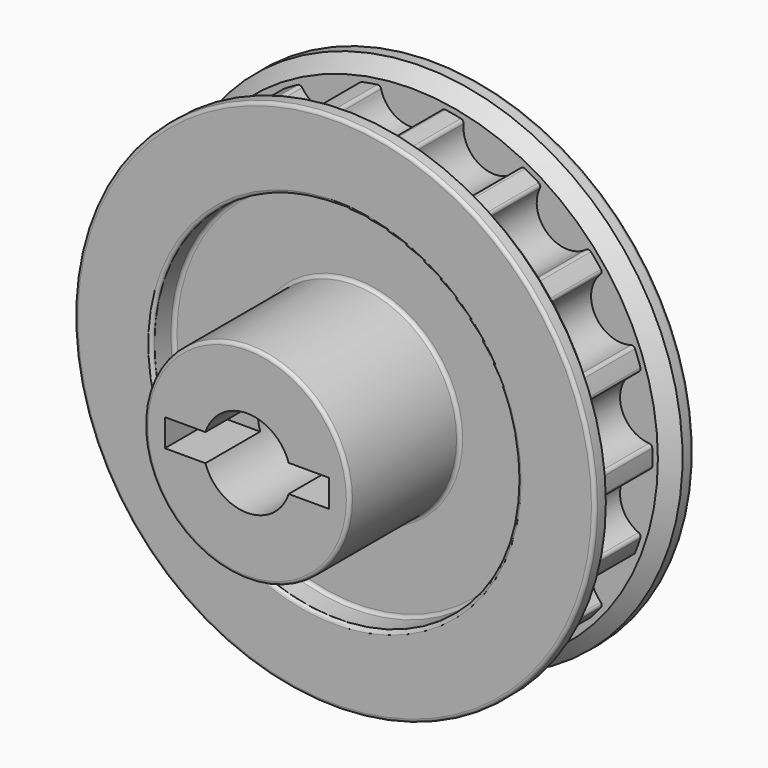
from build123d import *

# Parameters (mm, degrees)
F0_R      = 20.2099238274
F0_R_2    = 2.2772854034
F1_DEPTH  = 5
F2_R      = 21.3644414185
F2_R_2    = 17.5995160556
F3_DEPTH  = 5
F4_R      = 19
F4_R_2    = 13.3671533493
F5_DEPTH  = 2
F6_SIZE2  = 1
F6_SIZE   = 1
F7_R      = 19
F7_R_2    = 13.3703320349
F8_DEPTH  = 2
F9_SIZE2  = 1
F9_SIZE   = 1
F10_R     = 7.5
F11_DEPTH = 10
F12_R     = 3.2
F13_DEPTH = 15
F15_DEPTH = 5
F16_R     = 0.25


# Not quite as in the source:
# - two fillets or chamfers of one size are made in one step


with BuildPart() as f1:
    # F0 (on Front) → F1 (new body)
    with BuildSketch(Plane.XZ):
        with Locations((-33.3708077669, 18.9050808549)):
            Circle(F0_R)
        with Locations((-44.8001539134, 5.2841165238)):
            Circle(F0_R_2, mode=Mode.SUBTRACT)
        with Locations((-39.4522358284, 2.1964945778)):
            Circle(F0_R_2, mode=Mode.SUBTRACT)
        with Locations((-48.7695241739, 10.0146277921)):
            Circle(F0_R_2, mode=Mode.SUBTRACT)
        with Locations((-50.8815819749, 15.8174589089)):
            Circle(F0_R_2, mode=Mode.SUBTRACT)
        with Locations((-33.3708077669, 1.1241747293)):
            Circle(F0_R_2, mode=Mode.SUBTRACT)
        with Locations((-27.2893797054, 2.1964945778)):
            Circle(F0_R_2, mode=Mode.SUBTRACT)
        with Locations((-21.9414616204, 5.2841165238)):
            Circle(F0_R_2, mode=Mode.SUBTRACT)
        with Locations((-17.9720913599, 10.0146277921)):
            Circle(F0_R_2, mode=Mode.SUBTRACT)
        with Locations((-15.8600335589, 15.8174589089)):
            Circle(F0_R_2, mode=Mode.SUBTRACT)
        with Locations((-50.8815819749, 21.9927028009)):
            Circle(F0_R_2, mode=Mode.SUBTRACT)
        with Locations((-48.7695241739, 27.7955339177)):
            Circle(F0_R_2, mode=Mode.SUBTRACT)
        with Locations((-44.8001539134, 32.526045186)):
            Circle(F0_R_2, mode=Mode.SUBTRACT)
        with Locations((-39.4522358284, 35.613667132)):
            Circle(F0_R_2, mode=Mode.SUBTRACT)
        with Locations((-33.3708077669, 36.6859869804)):
            Circle(F0_R_2, mode=Mode.SUBTRACT)
        with Locations((-15.8600335589, 21.9927028009)):
            Circle(F0_R_2, mode=Mode.SUBTRACT)
        with Locations((-17.9720913599, 27.7955339177)):
            Circle(F0_R_2, mode=Mode.SUBTRACT)
        with Locations((-27.2893797054, 35.613667132)):
            Circle(F0_R_2, mode=Mode.SUBTRACT)
        with Locations((-21.9414616204, 32.526045186)):
            Circle(F0_R_2, mode=Mode.SUBTRACT)
    extrude(amount=F1_DEPTH)

    # F2 (on face) → F3 (cut)
    with BuildSketch(Plane.XZ.offset(5)):
        with Locations((-33.3708077669, 18.9050808549)):
            Circle(F2_R)
        with Locations((-33.3708077669, 18.9050808549)):
            Circle(F2_R_2, mode=Mode.SUBTRACT)
    extrude(amount=-F3_DEPTH, mode=Mode.SUBTRACT)

    # F4 (on face) → F5 (join)
    with BuildSketch(Plane.XZ.offset(5)):
        with Locations((-33.3708077669, 18.9050808549)):
            Circle(F4_R)
        with BuildLine():
            ThreePointArc((-46.3169163653, 6.982780844), (-46.8528192429, 7.5923299979), (-47.3600494173, 8.2259384063))
            ThreePointArc((-47.3600494173, 8.2259384063), (-46.797337163, 11.1532704938), (-49.6138372432, 12.1296134302))
            ThreePointArc((-49.6138372432, 12.1296134302), (-49.9089431338, 12.8856918511), (-50.1688767471, 13.654571934))
            ThreePointArc((-50.1688767471, 13.654571934), (-48.6388936539, 16.2129053692), (-50.9516090447, 18.0936673831))
            ThreePointArc((-50.9516090447, 18.0936673831), (-50.9703238225, 18.9050808549), (-50.9516090447, 19.7164943267))
            ThreePointArc((-50.9516090447, 19.7164943267), (-48.6388936539, 21.5972563405), (-50.1688767471, 24.1555897758))
            ThreePointArc((-50.1688767471, 24.1555897758), (-49.9089431338, 24.9244698587), (-49.6138372432, 25.6805482796))
            ThreePointArc((-49.6138372432, 25.6805482796), (-46.797337163, 26.656891216), (-47.3600494173, 29.5842233035))
            ThreePointArc((-47.3600494173, 29.5842233035), (-46.8528192429, 30.2178317119), (-46.3169163653, 30.8273808658))
            ThreePointArc((-46.3169163653, 30.8273808658), (-43.3363430724, 30.7815433574), (-42.8639130854, 33.7247946444))
            ThreePointArc((-42.8639130854, 33.7247946444), (-42.1705657947, 34.1467088533), (-41.4585037262, 34.5362081162))
            ThreePointArc((-41.4585037262, 34.5362081162), (-38.6733583484, 33.473718843), (-37.2227681487, 36.0778897867))
            ThreePointArc((-37.2227681487, 36.0778897867), (-36.4269316578, 36.2372207157), (-35.6245955928, 36.3596907281))
            ThreePointArc((-35.6245955928, 36.3596907281), (-33.3708077669, 34.4087015771), (-31.117019941, 36.3596907281))
            ThreePointArc((-31.117019941, 36.3596907281), (-30.314683876, 36.2372207157), (-29.5188473852, 36.0778897867))
            ThreePointArc((-29.5188473852, 36.0778897867), (-28.0682571854, 33.473718843), (-25.2831118076, 34.5362081162))
            ThreePointArc((-25.2831118076, 34.5362081162), (-24.5710497391, 34.1467088533), (-23.8777024485, 33.7247946444))
            ThreePointArc((-23.8777024485, 33.7247946444), (-23.4052724614, 30.7815433574), (-20.4246991685, 30.8273808658))
            ThreePointArc((-20.4246991685, 30.8273808658), (-19.8887962909, 30.2178317119), (-19.3815661165, 29.5842233035))
            ThreePointArc((-19.3815661165, 29.5842233035), (-19.9442783709, 26.656891216), (-17.1277782906, 25.6805482796))
            ThreePointArc((-17.1277782906, 25.6805482796), (-16.8326724001, 24.9244698587), (-16.5727387868, 24.1555897758))
            ThreePointArc((-16.5727387868, 24.1555897758), (-18.1027218799, 21.5972563405), (-15.7900064891, 19.7164943267))
            ThreePointArc((-15.7900064891, 19.7164943267), (-15.7712917113, 18.9050808549), (-15.7900064891, 18.0936673831))
            ThreePointArc((-15.7900064891, 18.0936673831), (-18.1027218799, 16.2129053692), (-16.5727387868, 13.654571934))
            ThreePointArc((-16.5727387868, 13.654571934), (-16.8326724001, 12.8856918511), (-17.1277782906, 12.1296134302))
            ThreePointArc((-17.1277782906, 12.1296134302), (-19.9442783709, 11.1532704938), (-19.3815661165, 8.2259384063))
            ThreePointArc((-19.3815661165, 8.2259384063), (-19.8887962909, 7.5923299979), (-20.4246991685, 6.982780844))
            ThreePointArc((-20.4246991685, 6.982780844), (-23.4052724614, 7.0286183524), (-23.8777024485, 4.0853670654))
            ThreePointArc((-23.8777024485, 4.0853670654), (-24.5710497391, 3.6634528564), (-25.2831118076, 3.2739535935))
            ThreePointArc((-25.2831118076, 3.2739535935), (-28.0682571854, 4.3364428668), (-29.5188473852, 1.7322719231))
            ThreePointArc((-29.5188473852, 1.7322719231), (-30.314683876, 1.5729409941), (-31.117019941, 1.4504709817))
            ThreePointArc((-31.117019941, 1.4504709817), (-33.3708077669, 3.4014601327), (-35.6245955928, 1.4504709817))
            ThreePointArc((-35.6245955928, 1.4504709817), (-36.4269316578, 1.5729409941), (-37.2227681487, 1.7322719231))
            ThreePointArc((-37.2227681487, 1.7322719231), (-38.6733583484, 4.3364428668), (-41.4585037262, 3.2739535935))
            ThreePointArc((-41.4585037262, 3.2739535935), (-42.1705657947, 3.6634528564), (-42.8639130854, 4.0853670654))
            ThreePointArc((-42.8639130854, 4.0853670654), (-43.3363430724, 7.0286183524), (-46.3169163653, 6.982780844))
        make_face(mode=Mode.SUBTRACT)
        with BuildLine():
            ThreePointArc((-49.6138372432, 12.1296134302), (-46.797337163, 11.1532704938), (-47.3600494173, 8.2259384063))
            ThreePointArc((-47.3600494173, 8.2259384063), (-46.8528192429, 7.5923299979), (-46.3169163653, 6.982780844))
            ThreePointArc((-46.3169163653, 6.982780844), (-43.3363430724, 7.0286183524), (-42.8639130854, 4.0853670654))
            ThreePointArc((-42.8639130854, 4.0853670654), (-42.1705657947, 3.6634528564), (-41.4585037262, 3.2739535935))
            ThreePointArc((-41.4585037262, 3.2739535935), (-38.6733583484, 4.3364428668), (-37.2227681487, 1.7322719231))
            ThreePointArc((-37.2227681487, 1.7322719231), (-36.4269316578, 1.5729409941), (-35.6245955928, 1.4504709817))
            ThreePointArc((-35.6245955928, 1.4504709817), (-33.3708077669, 3.4014601327), (-31.117019941, 1.4504709817))
            ThreePointArc((-31.117019941, 1.4504709817), (-30.314683876, 1.5729409941), (-29.5188473852, 1.7322719231))
            ThreePointArc((-29.5188473852, 1.7322719231), (-28.0682571854, 4.3364428668), (-25.2831118076, 3.2739535935))
            ThreePointArc((-25.2831118076, 3.2739535935), (-24.5710497391, 3.6634528564), (-23.8777024485, 4.0853670654))
            ThreePointArc((-23.8777024485, 4.0853670654), (-23.4052724614, 7.0286183524), (-20.4246991685, 6.982780844))
            ThreePointArc((-20.4246991685, 6.982780844), (-19.8887962909, 7.5923299979), (-19.3815661165, 8.2259384063))
            ThreePointArc((-19.3815661165, 8.2259384063), (-19.9442783709, 11.1532704938), (-17.1277782906, 12.1296134302))
            ThreePointArc((-17.1277782906, 12.1296134302), (-16.8326724001, 12.8856918511), (-16.5727387868, 13.654571934))
            ThreePointArc((-16.5727387868, 13.654571934), (-18.1027218799, 16.2129053692), (-15.7900064891, 18.0936673831))
            ThreePointArc((-15.7900064891, 18.0936673831), (-15.7712917113, 18.9050808549), (-15.7900064891, 19.7164943267))
            ThreePointArc((-15.7900064891, 19.7164943267), (-18.1027218799, 21.5972563405), (-16.5727387868, 24.1555897758))
            ThreePointArc((-16.5727387868, 24.1555897758), (-16.8326724001, 24.9244698587), (-17.1277782906, 25.6805482796))
            ThreePointArc((-17.1277782906, 25.6805482796), (-19.9442783709, 26.656891216), (-19.3815661165, 29.5842233035))
            ThreePointArc((-19.3815661165, 29.5842233035), (-19.8887962909, 30.2178317119), (-20.4246991685, 30.8273808658))
            ThreePointArc((-20.4246991685, 30.8273808658), (-23.4052724614, 30.7815433574), (-23.8777024485, 33.7247946444))
            ThreePointArc((-23.8777024485, 33.7247946444), (-24.5710497391, 34.1467088533), (-25.2831118076, 34.5362081162))
            ThreePointArc((-25.2831118076, 34.5362081162), (-28.0682571854, 33.473718843), (-29.5188473852, 36.0778897867))
            ThreePointArc((-29.5188473852, 36.0778897867), (-30.314683876, 36.2372207157), (-31.117019941, 36.3596907281))
            ThreePointArc((-31.117019941, 36.3596907281), (-33.3708077669, 34.4087015771), (-35.6245955928, 36.3596907281))
            ThreePointArc((-35.6245955928, 36.3596907281), (-36.4269316578, 36.2372207157), (-37.2227681487, 36.0778897867))
            ThreePointArc((-37.2227681487, 36.0778897867), (-38.6733583484, 33.473718843), (-41.4585037262, 34.5362081162))
            ThreePointArc((-41.4585037262, 34.5362081162), (-42.1705657947, 34.1467088533), (-42.8639130854, 33.7247946444))
            ThreePointArc((-42.8639130854, 33.7247946444), (-43.3363430724, 30.7815433574), (-46.3169163653, 30.8273808658))
            ThreePointArc((-46.3169163653, 30.8273808658), (-46.8528192429, 30.2178317119), (-47.3600494173, 29.5842233035))
            ThreePointArc((-47.3600494173, 29.5842233035), (-46.797337163, 26.656891216), (-49.6138372432, 25.6805482796))
            ThreePointArc((-49.6138372432, 25.6805482796), (-49.9089431338, 24.9244698587), (-50.1688767471, 24.1555897758))
            ThreePointArc((-50.1688767471, 24.1555897758), (-48.6388936539, 21.5972563405), (-50.9516090447, 19.7164943267))
            ThreePointArc((-50.9516090447, 19.7164943267), (-50.9703238225, 18.9050808549), (-50.9516090447, 18.0936673831))
            ThreePointArc((-50.9516090447, 18.0936673831), (-48.6388936539, 16.2129053692), (-50.1688767471, 13.654571934))
            ThreePointArc((-50.1688767471, 13.654571934), (-49.9089431338, 12.8856918511), (-49.6138372432, 12.1296134302))
        make_face()
        with Locations((-33.3708077669, 18.9050808549)):
            Circle(F4_R_2, mode=Mode.SUBTRACT)
    extrude(amount=F5_DEPTH)

    # F6
    f6_edges = [f1.edges().sort_by_distance(p)[0] for p in [
        (-52.370808, -5, 18.905081),
    ]]
    chamfer(f6_edges, length=F6_SIZE, length2=F6_SIZE2)

    # F7 (on face) → F8 (join)
    with BuildSketch(Plane(origin=(0, 0, 0), x_dir=(-1, 0, 0), z_dir=(0, 1, 0))):
        with Locations((33.3708077669, 18.9050808549)):
            Circle(F7_R)
        with BuildLine():
            ThreePointArc((47.3600494173, 8.2259384063), (46.8528192429, 7.5923299979), (46.3169163653, 6.982780844))
            ThreePointArc((46.3169163653, 6.982780844), (43.3363430724, 7.0286183524), (42.8639130854, 4.0853670654))
            ThreePointArc((42.8639130854, 4.0853670654), (42.1705657947, 3.6634528564), (41.4585037262, 3.2739535935))
            ThreePointArc((41.4585037262, 3.2739535935), (38.6733583484, 4.3364428668), (37.2227681487, 1.7322719231))
            ThreePointArc((37.2227681487, 1.7322719231), (36.4269316578, 1.5729409941), (35.6245955928, 1.4504709817))
            ThreePointArc((35.6245955928, 1.4504709817), (33.3708077669, 3.4014601327), (31.117019941, 1.4504709817))
            ThreePointArc((31.117019941, 1.4504709817), (30.314683876, 1.5729409941), (29.5188473852, 1.7322719231))
            ThreePointArc((29.5188473852, 1.7322719231), (28.0682571854, 4.3364428668), (25.2831118076, 3.2739535935))
            ThreePointArc((25.2831118076, 3.2739535935), (24.5710497391, 3.6634528564), (23.8777024485, 4.0853670654))
            ThreePointArc((23.8777024485, 4.0853670654), (23.4052724614, 7.0286183524), (20.4246991685, 6.982780844))
            ThreePointArc((20.4246991685, 6.982780844), (19.8887962909, 7.5923299979), (19.3815661165, 8.2259384063))
            ThreePointArc((19.3815661165, 8.2259384063), (19.9442783709, 11.1532704938), (17.1277782906, 12.1296134302))
            ThreePointArc((17.1277782906, 12.1296134302), (16.8326724001, 12.8856918511), (16.5727387868, 13.654571934))
            ThreePointArc((16.5727387868, 13.654571934), (18.1027218799, 16.2129053692), (15.7900064891, 18.0936673831))
            ThreePointArc((15.7900064891, 18.0936673831), (15.7712917113, 18.9050808549), (15.7900064891, 19.7164943267))
            ThreePointArc((15.7900064891, 19.7164943267), (18.1027218799, 21.5972563405), (16.5727387868, 24.1555897758))
            ThreePointArc((16.5727387868, 24.1555897758), (16.8326724001, 24.9244698587), (17.1277782906, 25.6805482796))
            ThreePointArc((17.1277782906, 25.6805482796), (19.9442783709, 26.656891216), (19.3815661165, 29.5842233035))
            ThreePointArc((19.3815661165, 29.5842233035), (19.8887962909, 30.2178317119), (20.4246991685, 30.8273808658))
            ThreePointArc((20.4246991685, 30.8273808658), (23.4052724614, 30.7815433574), (23.8777024485, 33.7247946444))
            ThreePointArc((23.8777024485, 33.7247946444), (24.5710497391, 34.1467088533), (25.2831118076, 34.5362081162))
            ThreePointArc((25.2831118076, 34.5362081162), (28.0682571854, 33.473718843), (29.5188473852, 36.0778897867))
            ThreePointArc((29.5188473852, 36.0778897867), (30.314683876, 36.2372207157), (31.117019941, 36.3596907281))
            ThreePointArc((31.117019941, 36.3596907281), (33.3708077669, 34.4087015771), (35.6245955928, 36.3596907281))
            ThreePointArc((35.6245955928, 36.3596907281), (36.4269316578, 36.2372207157), (37.2227681487, 36.0778897867))
            ThreePointArc((37.2227681487, 36.0778897867), (38.6733583484, 33.473718843), (41.4585037262, 34.5362081162))
            ThreePointArc((41.4585037262, 34.5362081162), (42.1705657947, 34.1467088533), (42.8639130854, 33.7247946444))
            ThreePointArc((42.8639130854, 33.7247946444), (43.3363430724, 30.7815433574), (46.3169163653, 30.8273808658))
            ThreePointArc((46.3169163653, 30.8273808658), (46.8528192429, 30.2178317119), (47.3600494173, 29.5842233035))
            ThreePointArc((47.3600494173, 29.5842233035), (46.797337163, 26.656891216), (49.6138372432, 25.6805482796))
            ThreePointArc((49.6138372432, 25.6805482796), (49.9089431338, 24.9244698587), (50.1688767471, 24.1555897758))
            ThreePointArc((50.1688767471, 24.1555897758), (48.6388936539, 21.5972563405), (50.9516090447, 19.7164943267))
            ThreePointArc((50.9516090447, 19.7164943267), (50.9703238225, 18.9050808549), (50.9516090447, 18.0936673831))
            ThreePointArc((50.9516090447, 18.0936673831), (48.6388936539, 16.2129053692), (50.1688767471, 13.654571934))
            ThreePointArc((50.1688767471, 13.654571934), (49.9089431338, 12.8856918511), (49.6138372432, 12.1296134302))
            ThreePointArc((49.6138372432, 12.1296134302), (46.797337163, 11.1532704938), (47.3600494173, 8.2259384063))
        make_face(mode=Mode.SUBTRACT)
        with BuildLine():
            ThreePointArc((42.8639130854, 4.0853670654), (43.3363430724, 7.0286183524), (46.3169163653, 6.982780844))
            ThreePointArc((46.3169163653, 6.982780844), (46.8528192429, 7.5923299979), (47.3600494173, 8.2259384063))
            ThreePointArc((47.3600494173, 8.2259384063), (46.797337163, 11.1532704938), (49.6138372432, 12.1296134302))
            ThreePointArc((49.6138372432, 12.1296134302), (49.9089431338, 12.8856918511), (50.1688767471, 13.654571934))
            ThreePointArc((50.1688767471, 13.654571934), (48.6388936539, 16.2129053692), (50.9516090447, 18.0936673831))
            ThreePointArc((50.9516090447, 18.0936673831), (50.9703238225, 18.9050808549), (50.9516090447, 19.7164943267))
            ThreePointArc((50.9516090447, 19.7164943267), (48.6388936539, 21.5972563405), (50.1688767471, 24.1555897758))
            ThreePointArc((50.1688767471, 24.1555897758), (49.9089431338, 24.9244698587), (49.6138372432, 25.6805482796))
            ThreePointArc((49.6138372432, 25.6805482796), (46.797337163, 26.656891216), (47.3600494173, 29.5842233035))
            ThreePointArc((47.3600494173, 29.5842233035), (46.8528192429, 30.2178317119), (46.3169163653, 30.8273808658))
            ThreePointArc((46.3169163653, 30.8273808658), (43.3363430724, 30.7815433574), (42.8639130854, 33.7247946444))
            ThreePointArc((42.8639130854, 33.7247946444), (42.1705657947, 34.1467088533), (41.4585037262, 34.5362081162))
            ThreePointArc((41.4585037262, 34.5362081162), (38.6733583484, 33.473718843), (37.2227681487, 36.0778897867))
            ThreePointArc((37.2227681487, 36.0778897867), (36.4269316578, 36.2372207157), (35.6245955928, 36.3596907281))
            ThreePointArc((35.6245955928, 36.3596907281), (33.3708077669, 34.4087015771), (31.117019941, 36.3596907281))
            ThreePointArc((31.117019941, 36.3596907281), (30.314683876, 36.2372207157), (29.5188473852, 36.0778897867))
            ThreePointArc((29.5188473852, 36.0778897867), (28.0682571854, 33.473718843), (25.2831118076, 34.5362081162))
            ThreePointArc((25.2831118076, 34.5362081162), (24.5710497391, 34.1467088533), (23.8777024485, 33.7247946444))
            ThreePointArc((23.8777024485, 33.7247946444), (23.4052724614, 30.7815433574), (20.4246991685, 30.8273808658))
            ThreePointArc((20.4246991685, 30.8273808658), (19.8887962909, 30.2178317119), (19.3815661165, 29.5842233035))
            ThreePointArc((19.3815661165, 29.5842233035), (19.9442783709, 26.656891216), (17.1277782906, 25.6805482796))
            ThreePointArc((17.1277782906, 25.6805482796), (16.8326724001, 24.9244698587), (16.5727387868, 24.1555897758))
            ThreePointArc((16.5727387868, 24.1555897758), (18.1027218799, 21.5972563405), (15.7900064891, 19.7164943267))
            ThreePointArc((15.7900064891, 19.7164943267), (15.7712917113, 18.9050808549), (15.7900064891, 18.0936673831))
            ThreePointArc((15.7900064891, 18.0936673831), (18.1027218799, 16.2129053692), (16.5727387868, 13.654571934))
            ThreePointArc((16.5727387868, 13.654571934), (16.8326724001, 12.8856918511), (17.1277782906, 12.1296134302))
            ThreePointArc((17.1277782906, 12.1296134302), (19.9442783709, 11.1532704938), (19.3815661165, 8.2259384063))
            ThreePointArc((19.3815661165, 8.2259384063), (19.8887962909, 7.5923299979), (20.4246991685, 6.982780844))
            ThreePointArc((20.4246991685, 6.982780844), (23.4052724614, 7.0286183524), (23.8777024485, 4.0853670654))
            ThreePointArc((23.8777024485, 4.0853670654), (24.5710497391, 3.6634528564), (25.2831118076, 3.2739535935))
            ThreePointArc((25.2831118076, 3.2739535935), (28.0682571854, 4.3364428668), (29.5188473852, 1.7322719231))
            ThreePointArc((29.5188473852, 1.7322719231), (30.314683876, 1.5729409941), (31.117019941, 1.4504709817))
            ThreePointArc((31.117019941, 1.4504709817), (33.3708077669, 3.4014601327), (35.6245955928, 1.4504709817))
            ThreePointArc((35.6245955928, 1.4504709817), (36.4269316578, 1.5729409941), (37.2227681487, 1.7322719231))
            ThreePointArc((37.2227681487, 1.7322719231), (38.6733583484, 4.3364428668), (41.4585037262, 3.2739535935))
            ThreePointArc((41.4585037262, 3.2739535935), (42.1705657947, 3.6634528564), (42.8639130854, 4.0853670654))
        make_face()
        with Locations((33.3708077669, 18.9050808549)):
            Circle(F7_R_2, mode=Mode.SUBTRACT)
    extrude(amount=F8_DEPTH)

    # F9
    f9_edges = [f1.edges().sort_by_distance(p)[0] for p in [
        (-14.370808, 0, 18.905081),
    ]]
    chamfer(f9_edges, length=F9_SIZE, length2=F9_SIZE2)

    # F10 (on face) → F11 (join)
    with BuildSketch(Plane.XZ.offset(5)):
        with Locations((-33.3708077669, 18.9050808549)):
            Circle(F10_R)
    extrude(amount=F11_DEPTH)

    # F12 (on face) → F13 (cut)
    with BuildSketch(Plane.XZ.offset(15)):
        with Locations((-33.3708077669, 18.9050808549)):
            Circle(F12_R)
    extrude(amount=-F13_DEPTH, mode=Mode.SUBTRACT)

    # F14 (on face) → F15 (cut)
    with BuildSketch(Plane.XZ.offset(15)):
        with BuildLine():
            Line((-36.4105445976, 19.9050808549), (-39.3708077669, 19.9050808549))
            Line((-39.3708077669, 19.9050808549), (-39.3708077669, 17.9050808549))
            Line((-39.3708077669, 17.9050808549), (-36.4105445976, 17.9050808549))
            ThreePointArc((-36.4105445976, 17.9050808549), (-36.5708077669, 18.9050808549), (-36.4105445976, 19.9050808549))
        make_face()
        with BuildLine():
            Line((-27.3708077669, 19.9050808549), (-30.3310709362, 19.9050808549))
            ThreePointArc((-30.3310709362, 19.9050808549), (-30.2111275728, 19.4114612167), (-30.1708077669, 18.9050808549))
            ThreePointArc((-30.1708077669, 18.9050808549), (-30.2111275728, 18.3987004931), (-30.3310709362, 17.9050808549))
            Line((-30.3310709362, 17.9050808549), (-27.3708077669, 17.9050808549))
            Line((-27.3708077669, 17.9050808549), (-27.3708077669, 19.9050808549))
        make_face()
    extrude(amount=-F15_DEPTH, mode=Mode.SUBTRACT)

    # F16
    f16_edges = [f1.edges().sort_by_distance(p)[0] for p in [
        (-23.877702, -2.5, 4.085367),
        (-20.424699, -2.5, 6.982781),
        (-19.381566, -2.5, 8.225938),
        (-17.127778, -2.5, 12.129613),
        (-16.572739, -2.5, 13.654572),
        (-15.790006, -2.5, 18.093667),
        (-15.790006, -2.5, 19.716494),
        (-16.572739, -2.5, 24.15559),
        (-49.613837, -2.5, 12.129613),
        (-47.360049, -2.5, 8.225938),
        (-50.168877, -2.5, 13.654572),
        (-50.951609, -2.5, 18.093667),
        (-50.951609, -2.5, 19.716494),
        (-50.168877, -2.5, 24.15559),
        (-49.613837, -2.5, 25.680548),
        (-47.360049, -2.5, 29.584223),
        (-46.316916, -2.5, 30.827381),
        (-42.863913, -2.5, 33.724795),
        (-41.458504, -2.5, 34.536208),
        (-37.222768, -2.5, 36.07789),
        (-35.624596, -2.5, 36.359691),
        (-31.11702, -2.5, 36.359691),
        (-29.518847, -2.5, 36.07789),
        (-25.283112, -2.5, 34.536208),
        (-23.877702, -2.5, 33.724795),
        (-20.424699, -2.5, 30.827381),
        (-19.381566, -2.5, 29.584223),
        (-17.127778, -2.5, 25.680548),
        (-25.283112, -2.5, 3.273954),
        (-29.518847, -2.5, 1.732272),
        (-31.11702, -2.5, 1.450471),
        (-35.624596, -2.5, 1.450471),
        (-37.222768, -2.5, 1.732272),
        (-41.458504, -2.5, 3.273954),
        (-42.863913, -2.5, 4.085367),
        (-46.316916, -2.5, 6.982781),
        (-14.370808, 2, 18.905081),
        (-20.000476, 2, 18.905081),
        (-20.000476, 0, 18.905081),
        (-52.370808, -7, 18.905081),
        (-46.737961, -7, 18.905081),
        (-46.737961, -5, 18.905081),
        (-40.870808, -15, 18.905081),
        (-40.870808, -5, 18.905081),
    ]]
    fillet(f16_edges, radius=F16_R)


solid = f1.part
